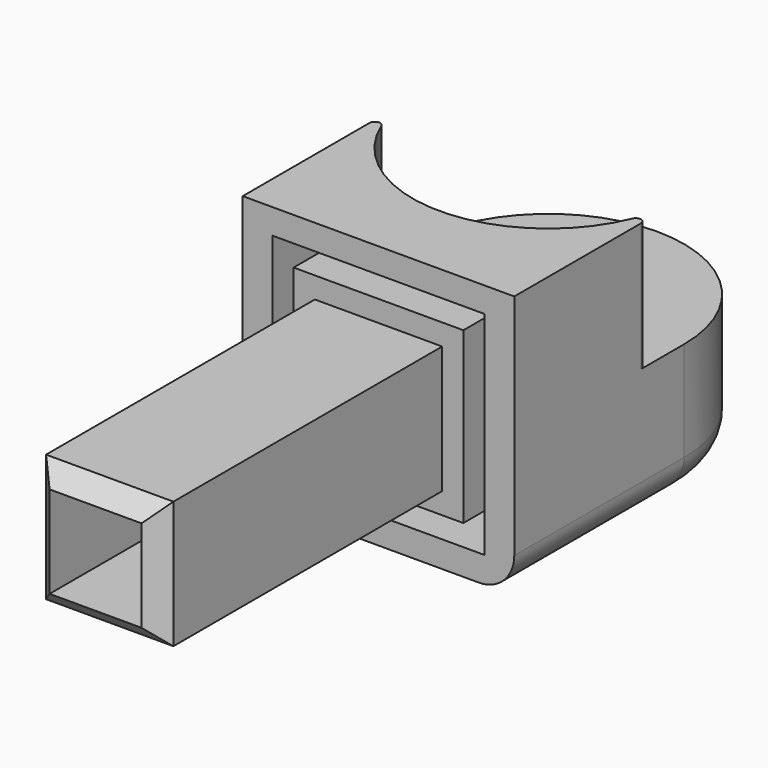
from build123d import *

# Parameters (mm, degrees)
F0_R     = 1.7145
F1_DEPTH = 9.7028
F2_DEPTH = 18.923
F3_F1_R  = 0.381
F3_F2_R  = 0.381
F4_W     = 9.144
F4_H     = 9.144
F5_DEPTH = 25.4
F6_SIZE  = 1.27
F8_DEPTH = 25.4
F4_W_2   = 15.24
F4_H_2   = 15.24
F4_W_3   = 12.192
F4_H_3   = 12.192
F9_DEPTH = 6.35
F10_R    = 2.54


with BuildPart() as f1:
    # F0 (on Top) → F1 (new body)
    with BuildSketch(Plane.XY):
        with BuildLine():
            ThreePointArc((-9.7536, 0), (0, -9.7536), (9.7536, 0))
            ThreePointArc((9.7536, 0), (0, 9.7536), (-9.7536, 0))
        make_face()
        Circle(F0_R, mode=Mode.SUBTRACT)
    extrude(amount=F1_DEPTH)

    # F0 (on Top) → F2 (join)
    with BuildSketch(Plane.XY):
        with BuildLine():
            Line((9.7536, -15.24), (9.7536, 0))
            ThreePointArc((9.7536, 0), (0, -9.7536), (-9.7536, 0))
            Line((-9.7536, 0), (-9.7536, -15.24))
            Line((-9.7536, -15.24), (9.7536, -15.24))
        make_face()
    extrude(amount=F2_DEPTH)

    # F3: fillet of radius 0.381 on 3 edges, made by hand

    # F3_f1
    f3_f1_edges = [f1.edges().sort_by_distance(p)[0] for p in [
        (9.7536, 0, 14.3129),
    ]]
    fillet(f3_f1_edges, radius=F3_F1_R)

    # F3_f2
    f3_f2_edges = [f1.edges().sort_by_distance(p)[0] for p in [
        (-9.7536, 0, 14.3129),
    ]]
    fillet(f3_f2_edges, radius=F3_F2_R)

    # F4 (on face) → F5 (join)
    with BuildSketch(Plane.XZ.offset(15.24)):
        with Locations((0, 9.500099346)):
            Rectangle(F4_W, F4_H)
    extrude(amount=F5_DEPTH)

    # F6
    f6_edges = [f1.edges().sort_by_distance(p)[0] for p in [
        (0, -40.64, 4.928099),
        (4.572, -40.64, 9.500099),
        (0, -40.64, 14.072099),
        (-4.572, -40.64, 9.500099),
    ]]
    chamfer(f6_edges, length=F6_SIZE)

    # F8 (cut): a face of the model
    f8_faces = [f1.faces().sort_by_distance(p)[0] for p in [
        (0, -40.64, 9.500099346),
    ]]
    extrude(f8_faces, amount=-F8_DEPTH, mode=Mode.SUBTRACT)

    # F4 (on face) → F9 (cut)
    with BuildSketch(Plane.XZ.offset(15.24)):
        with Locations((0, 9.500099346)):
            Rectangle(F4_W_2, F4_H_2)
        with Locations((0, 9.500099346)):
            Rectangle(F4_W_3, F4_H_3, mode=Mode.SUBTRACT)
    extrude(amount=-F9_DEPTH, mode=Mode.SUBTRACT)

    # F10
    f10_edges = [f1.edges().sort_by_distance(p)[0] for p in [
        (0, 9.7536, 0),
        (9.7536, -7.62, 0),
        (-9.7536, -7.62, 0),
    ]]
    fillet(f10_edges, radius=F10_R)


solid = f1.part
